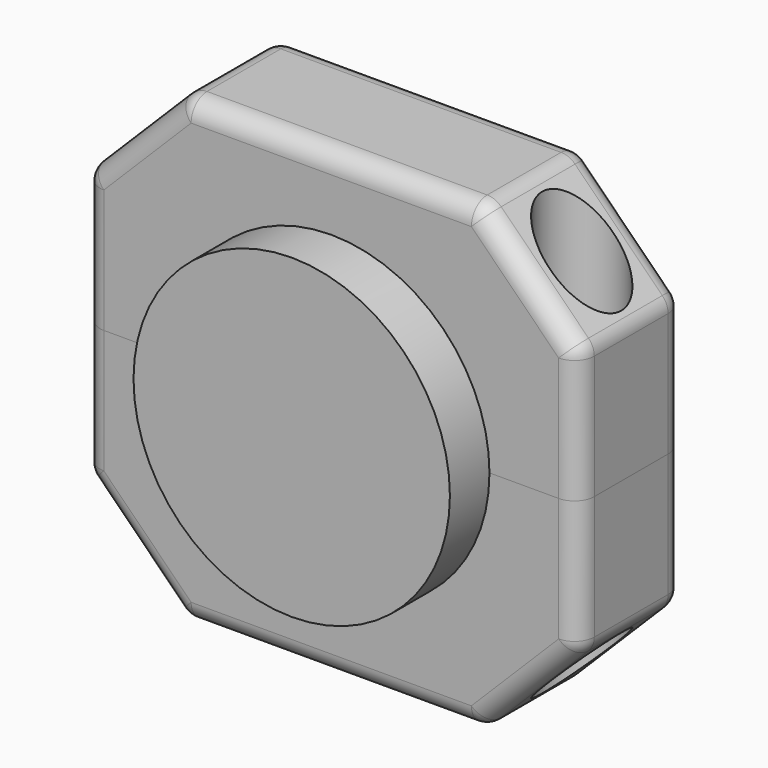
from build123d import *

# Parameters (mm, degrees)
F0_W          = 30
F0_H          = 20
F0_W_2        = 22.5
F1_DEPTH      = 35
F2_R          = 23.5
F3_DEPTH      = 25
F4_R          = 2
F5_DEPTH      = 25
F6_R          = 5
F7_DEPTH      = 29
F8_R          = 2
F9_DEPTH      = 35.001
F9_DEPTH_BACK = 107
F10_W         = 75
F10_H         = 20
F11_DEPTH     = 35
F12_R         = 23.5
F13_DEPTH     = 25
F14_R         = 2
F15_DEPTH     = 50
F16_R         = 6
F17_DEPTH     = 30
F18_T1_DEPTH  = 97.150489639
F19_T1_DEPTH  = 97.150489639
F20_R         = 24
F21_DEPTH     = 17.5
F22_R         = 3
F22_2_R       = 3
F23_R         = 6
F24_DEPTH     = 30


# Not quite as in the source:
# - a fillet or chamfer that OpenCascade refuses, or shapes differently, is made with other operations: its cross-section is extruded or revolved along the edge and cut away or added
# - an extrude ends at something that could not be found from the text; its depth is read off the source's solid
# - a feature names something its author has since deleted; it is built from what else it names


with BuildPart() as f1:
    # F0 (on Top) → F1 (new body)
    with BuildSketch(Plane.XY):
        Rectangle(F0_W, F0_H)
        with Locations((26.25, 0)):
            Rectangle(F0_W_2, F0_H)
        with Locations((-26.25, 0)):
            Rectangle(F0_W_2, F0_H)
    extrude(amount=F1_DEPTH)

    # F2 (on Front) → F3 (cut, symmetric)
    with BuildSketch(Plane.XZ):
        with Locations((0, 35)):
            Circle(F2_R)
    extrude(amount=F3_DEPTH, both=True, mode=Mode.SUBTRACT)

    # F4 (on face) → F5 (cut)
    with BuildSketch(Plane(origin=(0, 0, 0), x_dir=(1, 0, 0), z_dir=(0, 0, -1))):
        with Locations((7.75, 0)):
            Circle(F4_R)
        with Locations((-7.75, 0)):
            Circle(F4_R)
    extrude(amount=-F5_DEPTH, mode=Mode.SUBTRACT)

    # F6 (on face) → F7 (cut)
    with BuildSketch(Plane.XY.offset(35)):
        with Locations((7.75, 0)):
            Circle(F6_R)
        with Locations((-7.75, 0)):
            Circle(F6_R)
    extrude(amount=-F7_DEPTH, mode=Mode.SUBTRACT)

    # F8 (on face) → F9 (cut, two sides)
    with BuildSketch(Plane.XY.offset(35)) as f9_sk:
        with Locations((30, 0)):
            Circle(F8_R)
        with Locations((-30, 0)):
            Circle(F8_R)
    extrude(amount=-F9_DEPTH, mode=Mode.SUBTRACT)
    extrude(f9_sk.sketch, amount=F9_DEPTH_BACK, mode=Mode.SUBTRACT)

    # F19: chamfer of 15 on 2 edges, made by hand

    # F19_s2 → F19_t1 (cut)
    with BuildSketch(Plane.XZ.offset(-48.5752448195)):
        Polygon((37.5, 15), (22.5, 0), (37.5, 0), align=None)
        Polygon((-22.5, 0), (-37.5, 15), (-37.5, 0), align=None)
    extrude(amount=F19_T1_DEPTH, mode=Mode.SUBTRACT)

    # F22
    f22_edges = [f1.edges().sort_by_distance(p)[0] for p in [
        (37.5, -10, 25),
        (30, -10, 7.5),
        (37.5, 0, 15),
        (-37.5, -10, 25),
        (-30, -10, 7.5),
        (-37.5, 10, 25),
        (-30, 10, 7.5),
        (30, 10, 7.5),
        (37.5, 10, 25),
        (-37.5, 0, 15),
        (0, -10, 0),
        (0, 10, 0),
        (22.5, 0, 0),
        (-22.5, 0, 0),
    ]]
    fillet(f22_edges, radius=F22_R)

    # F23 (on face) → F24 (cut)
    with BuildSketch(Plane(origin=(0, 0, 0), x_dir=(1, 0, 0), z_dir=(0, 0, -1))):
        with Locations((30, 0)):
            Circle(F23_R)
        with Locations((-30, 0)):
            Circle(F23_R)
    extrude(amount=-F24_DEPTH, mode=Mode.SUBTRACT)


with BuildPart() as f11:
    # F10 (on face) → F11 (new body)
    with BuildSketch(Plane.XY.offset(35)):
        Rectangle(F10_W, F10_H)
    extrude(amount=F11_DEPTH)

    # F12 (on face) → F13 (cut, symmetric)
    with BuildSketch(Plane.XZ.offset(10)):
        with Locations((0, 35)):
            Circle(F12_R)
    extrude(amount=F13_DEPTH, both=True, mode=Mode.SUBTRACT)

    # F14 (on face) → F15 (cut)
    with BuildSketch(Plane.XY.offset(70)):
        with Locations((30, 0)):
            Circle(F14_R)
        with Locations((-30, 0)):
            Circle(F14_R)
    extrude(amount=-F15_DEPTH, mode=Mode.SUBTRACT)

    # F16 (on face) → F17 (cut)
    with BuildSketch(Plane.XY.offset(70)):
        with Locations((30, 0)):
            Circle(F16_R)
        with Locations((-30, 0)):
            Circle(F16_R)
    extrude(amount=-F17_DEPTH, mode=Mode.SUBTRACT)

    # F18: chamfer of 15 on 2 edges, made by hand

    # F18_s2 → F18_t1 (cut)
    with BuildSketch(Plane.XZ.offset(-48.5752448195)):
        Polygon((22.5, 70), (37.5, 55), (37.5, 70), align=None)
        Polygon((-37.5, 55), (-22.5, 70), (-37.5, 70), align=None)
    extrude(amount=F18_T1_DEPTH, mode=Mode.SUBTRACT)

    # F22#2
    f22_2_edges = [f11.edges().sort_by_distance(p)[0] for p in [
        (22.5, 0, 70),
        (37.5, 0, 55),
        (0, -10, 70),
        (30, -10, 62.5),
        (37.5, -10, 45),
        (-30, -10, 62.5),
        (-37.5, -10, 45),
        (30, 10, 62.5),
        (0, 10, 70),
        (-30, 10, 62.5),
        (-37.5, 10, 45),
        (37.5, 10, 45),
        (-37.5, 0, 55),
        (-22.5, 0, 70),
    ]]
    fillet(f22_2_edges, radius=F22_2_R)


with BuildPart() as f21:
    # F20 (on Front) → F21 (new body, symmetric)
    with BuildSketch(Plane.XZ):
        with Locations((0, 35)):
            Circle(F20_R)
    extrude(amount=F21_DEPTH, both=True)


solid = Compound([f1.part, f11.part, f21.part])
